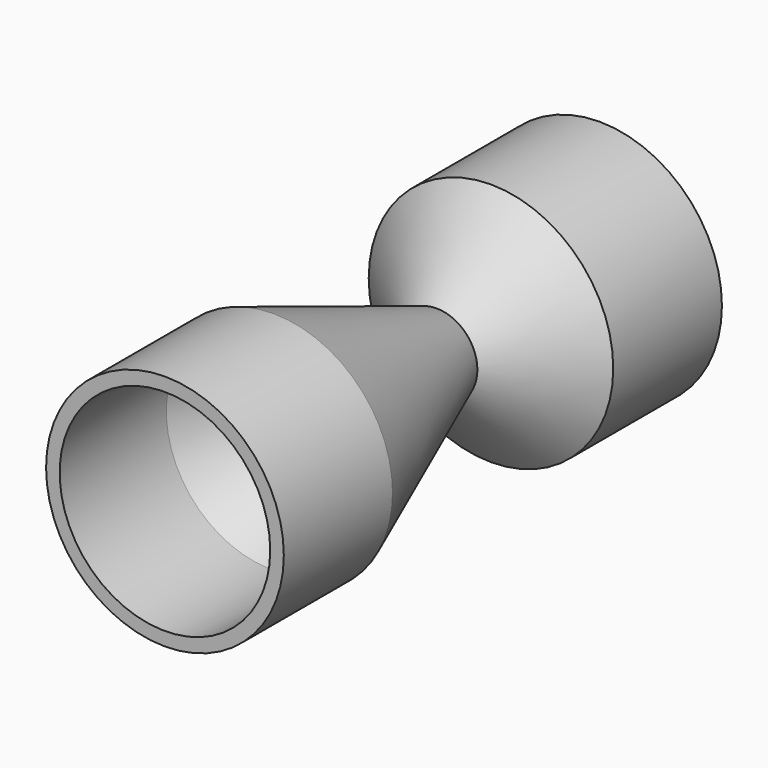
from build123d import *

# Parameters (mm, degrees)
F0_R         = 8.75
F4_R         = 3
F6_DEPTH     = 10
F10_R        = 9
F5_FACE1_R   = 3
F12_DEPTH    = 10
F13_T        = 1
F13_T4_ANGLE = 180.000000001
F13_T6_ANGLE = 180.000000001


# Not quite as in the source:
# - a shell that OpenCascade refuses in one call is made with other operations: the cavity is built on its own and cut out


with BuildPart() as f5:
    # F0 (on Front) → F5 section 0
    with BuildSketch(Plane.XZ):
        Circle(F0_R)
    # F4 (on line) → F5 section 1
    with BuildSketch(Plane(origin=(0, 15, 0), x_dir=(-1, 0, 0), z_dir=(0, 1, 0))):
        Circle(F4_R)
    loft()

    # F6 (add): a face of the model
    f6_faces = [f5.faces().sort_by_distance(p)[0] for p in [
        (0, 0, 0),
    ]]
    extrude(f6_faces, amount=F6_DEPTH)

    # F10 (on line) → F11 section 0
    with BuildSketch(Plane(origin=(0, 20, 0), x_dir=(-1, 0, 0), z_dir=(0, 1, 0))):
        Circle(F10_R)
    # F5_face1 (on face) → F11 section 1
    with BuildSketch(Plane(origin=(0, 15, 0), x_dir=(-1, 0, 0), z_dir=(0, 1, 0))):
        Circle(F5_FACE1_R)
    loft()

    # F12 (add): a face of the model
    f12_faces = [f5.faces().sort_by_distance(p)[0] for p in [
        (0, 20, 0),
    ]]
    extrude(f12_faces, amount=F12_DEPTH)

    # F13: shell of thickness 1, made by hand


with BuildPart() as f13_core1:
    # F13_t2: copy of F5
    add(f5.part)

    # the walls: a layer under each face that stays
    f13_faces = [f13_core1.faces().sort_by_distance(p)[0] for p in [
        (-5.875, 7.5, 0),
        (6, 17.5, 0),
        (-8.75, -5, 0),
        (9, 25, 0),
    ]]
    thicken(f13_faces, amount=-F13_T, mode=Mode.SUBTRACT)

    # F13_s3 → F13_t4 (revolve, cut)
    with BuildSketch(Plane.XY):
        Polygon((3.0157393052, 14.9958971473), (2.0662538827, 14.6420639884), (1.8101483908, 15.3101652716), (2.3598156003, 15.7682212796), align=None)
    revolve(axis=Axis((0, 15, 0), (0, -1, 0)), revolution_arc=F13_T4_ANGLE, mode=Mode.SUBTRACT)

    # F13_s5 → F13_t6 (revolve, cut)
    with BuildSketch(Plane.XY):
        Polygon((-3.0157393052, 14.9958971473), (-2.0662538827, 14.6420639884), (-1.8101483908, 15.3101652716), (-2.3598156003, 15.7682212796), align=None)
    revolve(axis=Axis((0, 15, 0), (0, -1, 0)), revolution_arc=F13_T6_ANGLE, mode=Mode.SUBTRACT)


with BuildPart() as f5_1:
    add(f5.part)

    # what is left inside the walls is the cavity
    f13_cavity = [f13_core1.part.solids().sort_by_distance(p)[0] for p in [
        (-5.84608, 4.753709, 0),
    ]]
    add(f13_cavity, mode=Mode.SUBTRACT)


solid = f5_1.part
